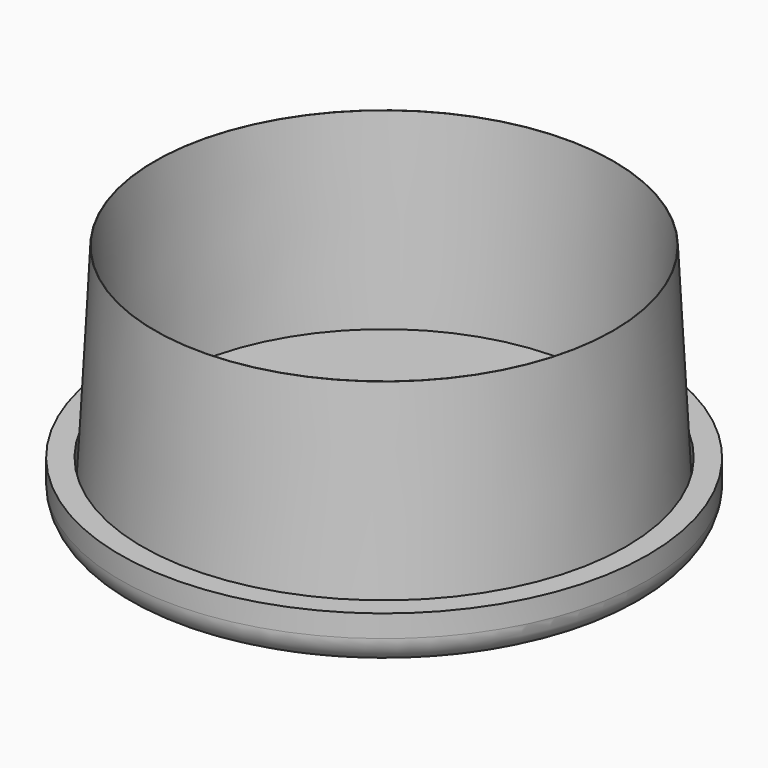
from build123d import *

# Parameters (mm, degrees)
F0_R     = 25.65
F0_R_2   = 23
F1_DEPTH = 25
F1_TAPER = 3
F2_DEPTH = 5.25
F0_R_3   = 28.0000000894
F3_DEPTH = 5.25


# Not quite as in the source:
# - a fillet or chamfer that OpenCascade refuses, or shapes differently, is made with other operations: its cross-section is extruded or revolved along the edge and cut away or added


with BuildPart() as f1:
    # F0 (on Top) → F1 (new body)
    with BuildSketch(Plane.XY):
        Circle(F0_R)
        Circle(F0_R_2, mode=Mode.SUBTRACT)
    extrude(amount=F1_DEPTH, taper=F1_TAPER)


with BuildPart() as f2:
    # F0 (on Top) → F2 (new body)
    with BuildSketch(Plane.XY):
        Circle(F0_R_2)
    extrude(amount=F2_DEPTH)


with BuildPart() as f3:
    # F0 (on Top) → F3 (new body)
    with BuildSketch(Plane.XY):
        Circle(F0_R_3)
        Circle(F0_R, mode=Mode.SUBTRACT)
    extrude(amount=F3_DEPTH)

    # F4: fillet of radius 3 on 1 edges, made by hand

    # F4_s1 → F4_t2 (revolve, cut)
    with BuildSketch(Plane.XZ):
        with BuildLine():
            ThreePointArc((28.0001500894, 2.9286165874), (27.3399841876, 1.0510712769), (25.6500324941, -0.0001464382))
            Line((25.6500324941, -0.0001464382), (25.6630301422, -0.0587216987))
            ThreePointArc((25.6630301422, -0.0587216987), (26.8250162918, -0.06), (28.0000000894, -0.06))
            Line((28.0000000894, -0.06), (28.0600000894, 0))
            ThreePointArc((28.0600000894, 0), (28.0600000894, 1.4643082937), (28.0601500894, 2.9286165874))
            Line((28.0601500894, 2.9286165874), (28.0001500894, 2.9286165874))
        make_face()
    revolve(axis=Axis((0, 0, 0), (0, 0, 1)), mode=Mode.SUBTRACT)


solid = Compound([f1.part, f2.part, f3.part])
